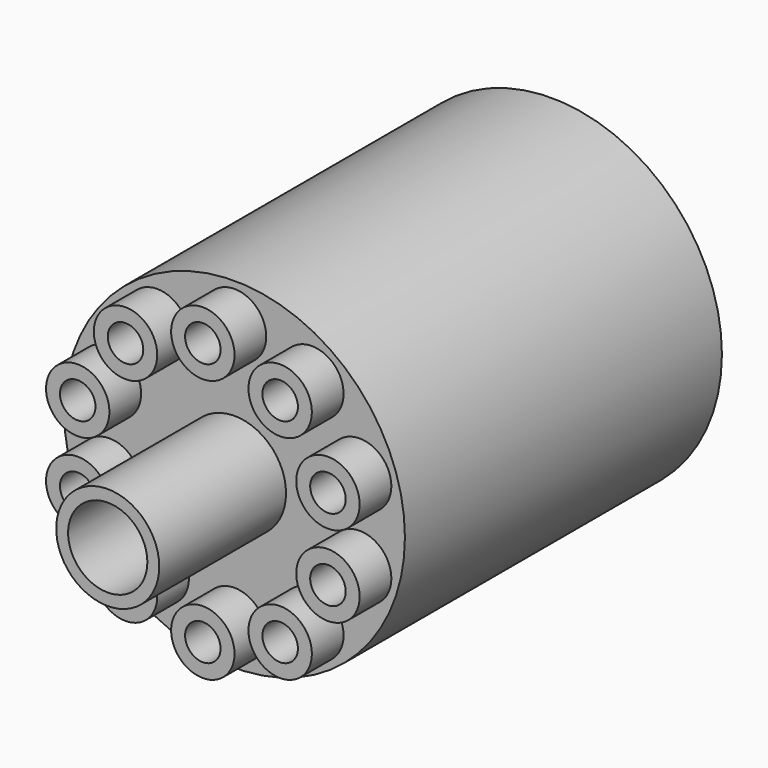
from build123d import *
from build123d import SkipClean  # not in build123d's __all__

# Parameters (mm, degrees)
F0_R     = 27.305
F1_DEPTH = 63.5
F3_DEPTH = 86.614
F4_R     = 5.08
F4_R_2   = 2.8448
F5_DEPTH = 6.35
F6_R     = 8.255
F6_R_2   = 6.35
F7_DEPTH = 25.4
F8_DEPTH = 36.5252
F9_DEPTH = 133.35


# Not quite as in the source:
# - after a boolean that leaves OpenCascade's solid faulty, fix() repairs it


with BuildPart() as f1:
    # F0 (on Front) → F1 (new body)
    with BuildSketch(Plane.XZ):
        Circle(F0_R)
    extrude(amount=F1_DEPTH)

    # F2 (on face) → F3 (cut)
    with BuildSketch(Plane(origin=(0, 0, 0), x_dir=(-1, 0, 0), z_dir=(0, 1, 0))):
        with BuildLine():
            ThreePointArc((-17.2053734765, -6.5146962754), (-17.2403976852, -6.0696715093), (-17.344607899, -5.6356047298))
            ThreePointArc((-17.344607899, -5.6356047298), (-22.8599492679, -6.9597210416), (-17.2053734765, -6.5146962754))
        make_face()
        with BuildLine():
            ThreePointArc((-17.2053734765, 6.5146962754), (-22.8599492679, 6.9597210416), (-17.344607899, 5.6356047298))
            ThreePointArc((-17.344607899, 5.6356047298), (-17.2403976852, 6.0696715093), (-17.2053734765, 6.5146962754))
        make_face()
        with BuildLine():
            ThreePointArc((-9.5468886888, 17.0556962754), (-14.9264240488, 18.3472084491), (-10.7195572031, 14.7542047298))
            ThreePointArc((-10.7195572031, 14.7542047298), (-9.8569533288, 15.7641841018), (-9.5468886888, 17.0556962754))
        make_face()
        with BuildLine():
            ThreePointArc((2.8448, 21.082), (-2.0115773711, 23.0935773711), (0, 18.2372))
            ThreePointArc((0, 18.2372), (2.0115773711, 19.0704226289), (2.8448, 21.082))
        make_face()
        with BuildLine():
            ThreePointArc((15.2364886888, 17.0556962754), (11.1001765152, 19.5904316354), (10.7195572031, 14.7542047298))
            ThreePointArc((10.7195572031, 14.7542047298), (13.6832008625, 14.5209609154), (15.2364886888, 17.0556962754))
        make_face()
        with BuildLine():
            ThreePointArc((22.8949734765, 6.5146962754), (19.6051487104, 9.3244720667), (17.344607899, 5.6356047298))
            ThreePointArc((17.344607899, 5.6356047298), (20.4951982427, 3.7049204841), (22.8949734765, 6.5146962754))
        make_face()
        with BuildLine():
            ThreePointArc((22.8949734765, -6.5146962754), (20.4951982427, -3.7049204841), (17.344607899, -5.6356047298))
            ThreePointArc((17.344607899, -5.6356047298), (19.6051487104, -9.3244720667), (22.8949734765, -6.5146962754))
        make_face()
        with BuildLine():
            ThreePointArc((15.2364886888, -17.0556962754), (13.6832008625, -14.5209609154), (10.7195572031, -14.7542047298))
            ThreePointArc((10.7195572031, -14.7542047298), (11.1001765152, -19.5904316354), (15.2364886888, -17.0556962754))
        make_face()
        with BuildLine():
            ThreePointArc((2.8448, -21.082), (2.0115773711, -19.0704226289), (0, -18.2372))
            ThreePointArc((0, -18.2372), (-2.0115773711, -23.0935773711), (2.8448, -21.082))
        make_face()
        with BuildLine():
            ThreePointArc((-9.5468886888, -17.0556962754), (-9.8569533288, -15.7641841018), (-10.7195572031, -14.7542047298))
            ThreePointArc((-10.7195572031, -14.7542047298), (-14.9264240488, -18.3472084491), (-9.5468886888, -17.0556962754))
        make_face()
    extrude(amount=-F3_DEPTH, mode=Mode.SUBTRACT)

    # F4 (on face) → F5 (join)
    with BuildSketch(Plane.XZ.offset(63.5)):
        with Locations((0, 21.082)):
            Circle(F4_R)
        with Locations((0, 21.082)):
            Circle(F4_R_2, mode=Mode.SUBTRACT)
        with Locations((12.3916886888, 17.0556962754)):
            Circle(F4_R)
        with Locations((12.3916886888, 17.0556962754)):
            Circle(F4_R_2, mode=Mode.SUBTRACT)
        with Locations((20.0501734765, 6.5146962754)):
            Circle(F4_R)
        with Locations((20.0501734765, 6.5146962754)):
            Circle(F4_R_2, mode=Mode.SUBTRACT)
        with Locations((20.0501734765, -6.5146962754)):
            Circle(F4_R)
        with Locations((20.0501734765, -6.5146962754)):
            Circle(F4_R_2, mode=Mode.SUBTRACT)
        with Locations((12.3916886888, -17.0556962754)):
            Circle(F4_R)
        with Locations((12.3916886888, -17.0556962754)):
            Circle(F4_R_2, mode=Mode.SUBTRACT)
        with Locations((0, -21.082)):
            Circle(F4_R)
        with Locations((0, -21.082)):
            Circle(F4_R_2, mode=Mode.SUBTRACT)
        with Locations((-12.3916886888, -17.0556962754)):
            Circle(F4_R)
        with Locations((-12.3916886888, -17.0556962754)):
            Circle(F4_R_2, mode=Mode.SUBTRACT)
        with Locations((-20.0501734765, -6.5146962754)):
            Circle(F4_R)
        with Locations((-20.0501734765, -6.5146962754)):
            Circle(F4_R_2, mode=Mode.SUBTRACT)
        with Locations((-20.0501734765, 6.5146962754)):
            Circle(F4_R)
        with Locations((-20.0501734765, 6.5146962754)):
            Circle(F4_R_2, mode=Mode.SUBTRACT)
        with Locations((-12.3916886888, 17.0556962754)):
            Circle(F4_R)
        with Locations((-12.3916886888, 17.0556962754)):
            Circle(F4_R_2, mode=Mode.SUBTRACT)
    with SkipClean():  # cleaning this boolean's faces spoils the solid; the shape is the same uncleaned
        extrude(amount=F5_DEPTH)

    # F6 (on face) → F7 (join)
    with BuildSketch(Plane.XZ.offset(63.5)):
        Circle(F6_R)
        Circle(F6_R_2, mode=Mode.SUBTRACT)
    extrude(amount=F7_DEPTH)

    add(f1.part.fix(), mode=Mode.REPLACE)

    # F2 (on face) → F8 (cut)
    with BuildSketch(Plane(origin=(0, 0, 0), x_dir=(-1, 0, 0), z_dir=(0, 1, 0))):
        with BuildLine():
            ThreePointArc((-7.6164886888, 17.0556962754), (-16.6464230431, 19.2235917098), (-9.5848965521, 13.1924783239))
            ThreePointArc((-9.5848965521, 13.1924783239), (-8.1369543345, 14.8878008411), (-7.6164886888, 17.0556962754))
        make_face()
        with BuildLine():
            ThreePointArc((-9.5468886888, 17.0556962754), (-9.8569533288, 15.7641841018), (-10.7195572031, 14.7542047298))
            ThreePointArc((-10.7195572031, 14.7542047298), (-14.9264240488, 18.3472084491), (-9.5468886888, 17.0556962754))
        make_face(mode=Mode.SUBTRACT)
        with BuildLine():
            ThreePointArc((4.7752, 21.082), (-3.3765763015, 24.4585763015), (0, 16.3068))
            ThreePointArc((0, 16.3068), (3.3765763015, 17.7054236985), (4.7752, 21.082))
        make_face()
        with BuildLine():
            ThreePointArc((2.8448, 21.082), (2.0115773711, 19.0704226289), (0, 18.2372))
            ThreePointArc((0, 18.2372), (-2.0115773711, 23.0935773711), (2.8448, 21.082))
        make_face(mode=Mode.SUBTRACT)
        with BuildLine():
            ThreePointArc((17.1668886888, 17.0556962754), (10.2237932545, 21.3104306297), (9.5848965521, 13.1924783239))
            ThreePointArc((9.5848965521, 13.1924783239), (14.5595841232, 12.8009619211), (17.1668886888, 17.0556962754))
        make_face()
        with BuildLine():
            ThreePointArc((15.2364886888, 17.0556962754), (13.6832008625, 14.5209609154), (10.7195572031, 14.7542047298))
            ThreePointArc((10.7195572031, 14.7542047298), (11.1001765152, 19.5904316354), (15.2364886888, 17.0556962754))
        make_face(mode=Mode.SUBTRACT)
        with BuildLine():
            ThreePointArc((24.8253734765, 6.5146962754), (19.3031676191, 11.2311056394), (15.5086883999, 5.0390783239))
            ThreePointArc((15.5086883999, 5.0390783239), (20.797179334, 1.7982869114), (24.8253734765, 6.5146962754))
        make_face()
        with BuildLine():
            ThreePointArc((22.8949734765, 6.5146962754), (20.4951982427, 3.7049204841), (17.344607899, 5.6356047298))
            ThreePointArc((17.344607899, 5.6356047298), (19.6051487104, 9.3244720667), (22.8949734765, 6.5146962754))
        make_face(mode=Mode.SUBTRACT)
        with BuildLine():
            ThreePointArc((24.8253734765, -6.5146962754), (20.797179334, -1.7982869114), (15.5086883999, -5.0390783239))
            ThreePointArc((15.5086883999, -5.0390783239), (19.3031676191, -11.2311056394), (24.8253734765, -6.5146962754))
        make_face()
        with BuildLine():
            ThreePointArc((22.8949734765, -6.5146962754), (19.6051487104, -9.3244720667), (17.344607899, -5.6356047298))
            ThreePointArc((17.344607899, -5.6356047298), (20.4951982427, -3.7049204841), (22.8949734765, -6.5146962754))
        make_face(mode=Mode.SUBTRACT)
        with BuildLine():
            ThreePointArc((17.1668886888, -17.0556962754), (14.5595841232, -12.8009619211), (9.5848965521, -13.1924783239))
            ThreePointArc((9.5848965521, -13.1924783239), (10.2237932545, -21.3104306297), (17.1668886888, -17.0556962754))
        make_face()
        with BuildLine():
            ThreePointArc((15.2364886888, -17.0556962754), (11.1001765152, -19.5904316354), (10.7195572031, -14.7542047298))
            ThreePointArc((10.7195572031, -14.7542047298), (13.6832008625, -14.5209609154), (15.2364886888, -17.0556962754))
        make_face(mode=Mode.SUBTRACT)
        with BuildLine():
            ThreePointArc((4.7752, -21.082), (3.3765763015, -17.7054236985), (0, -16.3068))
            ThreePointArc((0, -16.3068), (-3.3765763015, -24.4585763015), (4.7752, -21.082))
        make_face()
        with BuildLine():
            ThreePointArc((2.8448, -21.082), (-2.0115773711, -23.0935773711), (0, -18.2372))
            ThreePointArc((0, -18.2372), (2.0115773711, -19.0704226289), (2.8448, -21.082))
        make_face(mode=Mode.SUBTRACT)
        with BuildLine():
            ThreePointArc((-7.6164886888, -17.0556962754), (-8.1369543345, -14.8878008411), (-9.5848965521, -13.1924783239))
            ThreePointArc((-9.5848965521, -13.1924783239), (-16.6464230431, -19.2235917098), (-7.6164886888, -17.0556962754))
        make_face()
        with BuildLine():
            ThreePointArc((-9.5468886888, -17.0556962754), (-14.9264240488, -18.3472084491), (-10.7195572031, -14.7542047298))
            ThreePointArc((-10.7195572031, -14.7542047298), (-9.8569533288, -15.7641841018), (-9.5468886888, -17.0556962754))
        make_face(mode=Mode.SUBTRACT)
        with BuildLine():
            ThreePointArc((-15.2749734765, -6.5146962754), (-15.3337641125, -5.767690418), (-15.5086883999, -5.0390783239))
            ThreePointArc((-15.5086883999, -5.0390783239), (-24.7665828405, -7.2617021329), (-15.2749734765, -6.5146962754))
        make_face()
        with BuildLine():
            ThreePointArc((-17.2053734765, -6.5146962754), (-22.8599492679, -6.9597210416), (-17.344607899, -5.6356047298))
            ThreePointArc((-17.344607899, -5.6356047298), (-17.2403976852, -6.0696715093), (-17.2053734765, -6.5146962754))
        make_face(mode=Mode.SUBTRACT)
        with BuildLine():
            ThreePointArc((-15.2749734765, 6.5146962754), (-24.7665828405, 7.2617021329), (-15.5086883999, 5.0390783239))
            ThreePointArc((-15.5086883999, 5.0390783239), (-15.3337641125, 5.767690418), (-15.2749734765, 6.5146962754))
        make_face()
        with BuildLine():
            ThreePointArc((-17.2053734765, 6.5146962754), (-17.2403976852, 6.0696715093), (-17.344607899, 5.6356047298))
            ThreePointArc((-17.344607899, 5.6356047298), (-22.8599492679, 6.9597210416), (-17.2053734765, 6.5146962754))
        make_face(mode=Mode.SUBTRACT)
    extrude(amount=-F8_DEPTH, mode=Mode.SUBTRACT)

    add(f1.part.fix(), mode=Mode.REPLACE)

    # F9 (cut): a face of the model
    f9_faces = [f1.faces().sort_by_distance(p)[0] for p in [
        (0, -63.5, 0),
    ]]
    extrude(f9_faces, amount=-F9_DEPTH, mode=Mode.SUBTRACT)


solid = f1.part
